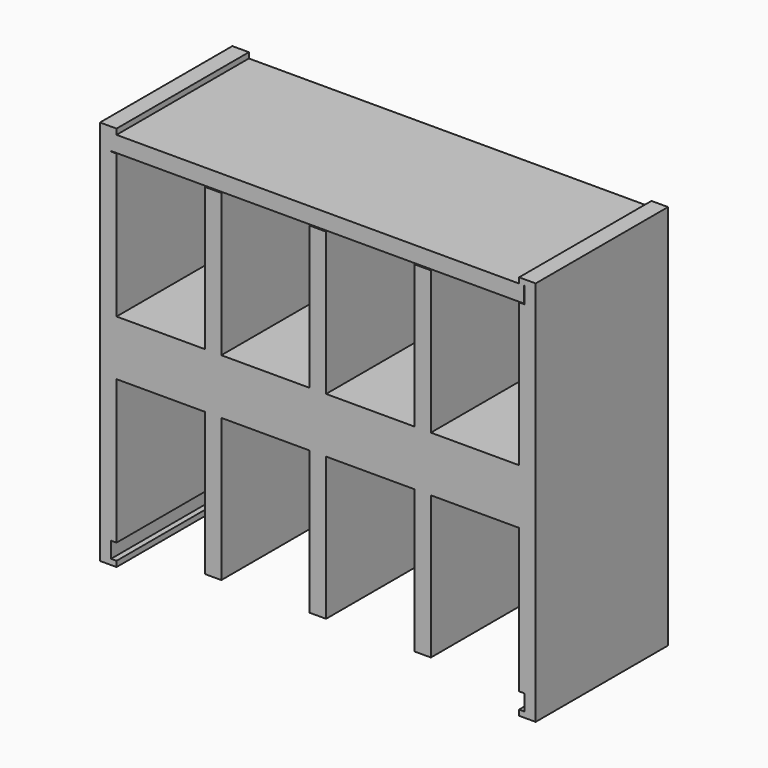
from build123d import *

# Parameters (mm, degrees)
F0_W      = 39.5
F0_H      = 15
F1_DEPTH  = 5
F2_W      = 1.5
F2_H      = 15
F3_DEPTH  = 15
F5_W      = 1.5
F5_H      = 15
F6_DEPTH  = 15
F7_DEPTH  = 12.95
F9_W      = 0.5
F9_H      = 1.5
F10_DEPTH = 15
F9_W_2    = 1.5
F9_H_2    = 2.05
F9_H_3    = 2.0491243154
F11_DEPTH = 15
F13_DEPTH = 15
F14_W     = 0.5
F14_H     = 1.45
F15_DEPTH = 15


# Not quite as in the source:
# - the program builds the solid bodies; features that only make, move or delete a surface that nothing else refers to are left out


with BuildPart() as f1:
    # F0 (on Top) → F1 (new body)
    with BuildSketch(Plane.XY):
        Rectangle(F0_W, F0_H)
    extrude(amount=F1_DEPTH)

    # F2 (on face) → F3 (join)
    with BuildSketch(Plane.XY.offset(5)):
        with Locations((-19, 0)):
            Rectangle(F2_W, F2_H)
        with Locations((-9.5, 0)):
            Rectangle(F2_W, F2_H)
        Rectangle(F2_W, F2_H)
        with Locations((9.5, 0)):
            Rectangle(F2_W, F2_H)
        with Locations((19, 0)):
            Rectangle(F2_W, F2_H)
    extrude(amount=F3_DEPTH)

    # F5 (on face) → F6 (join)
    with BuildSketch(Plane(origin=(0, 0, 0), x_dir=(1, 0, 0), z_dir=(0, 0, -1))):
        with Locations((-19, 0)):
            Rectangle(F5_W, F5_H)
        with Locations((19, 0)):
            Rectangle(F5_W, F5_H)
    extrude(amount=F6_DEPTH)

    # F5 (on face) → F7 (join)
    with BuildSketch(Plane(origin=(0, 0, 0), x_dir=(1, 0, 0), z_dir=(0, 0, -1))):
        with Locations((-9.5, 0)):
            Rectangle(F5_W, F5_H)
        Rectangle(F5_W, F5_H)
        with Locations((9.5, 0)):
            Rectangle(F5_W, F5_H)
    extrude(amount=F7_DEPTH)

    # F9 (on face) → F10 (cut)
    with BuildSketch(Plane(origin=(0, 7.5, 0), x_dir=(-1, 0, 0), z_dir=(0, 1, 0))):
        with Locations((18.5, 18.75)):
            Rectangle(F9_W, F9_H)
        with Locations((-18.5, 18.75)):
            Rectangle(F9_W, F9_H)
    extrude(amount=-F10_DEPTH, mode=Mode.SUBTRACT)

    # F9 (on face) → F11 (cut)
    with BuildSketch(Plane(origin=(0, 7.5, 0), x_dir=(-1, 0, 0), z_dir=(0, 1, 0))):
        with Locations((-9.5, 18.975)):
            Rectangle(F9_W_2, F9_H_2)
        with Locations((0, 18.9754378423)):
            Rectangle(F9_W_2, F9_H_3)
        with Locations((9.5, 18.9754378423)):
            Rectangle(F9_W_2, F9_H_3)
    extrude(amount=-F11_DEPTH, mode=Mode.SUBTRACT)

    # F12 (on face) → F13 (join)
    with BuildSketch(Plane.XZ.offset(7.5)):
        Polygon((-18.25, 19.5), (-18.75, 19.5), (-18.75, 18.05), (18.7, 18.05), (18.7, 19.5), (18.25, 19.5), align=None)
    extrude(amount=-F13_DEPTH)

    # F14 (on face) → F15 (cut)
    with BuildSketch(Plane.XZ.offset(7.5)):
        with Locations((18.5, -13.775)):
            Rectangle(F14_W, F14_H)
        with Locations((-18.5, -13.775)):
            Rectangle(F14_W, F14_H)
    extrude(amount=-F15_DEPTH, mode=Mode.SUBTRACT)


solid = f1.part
